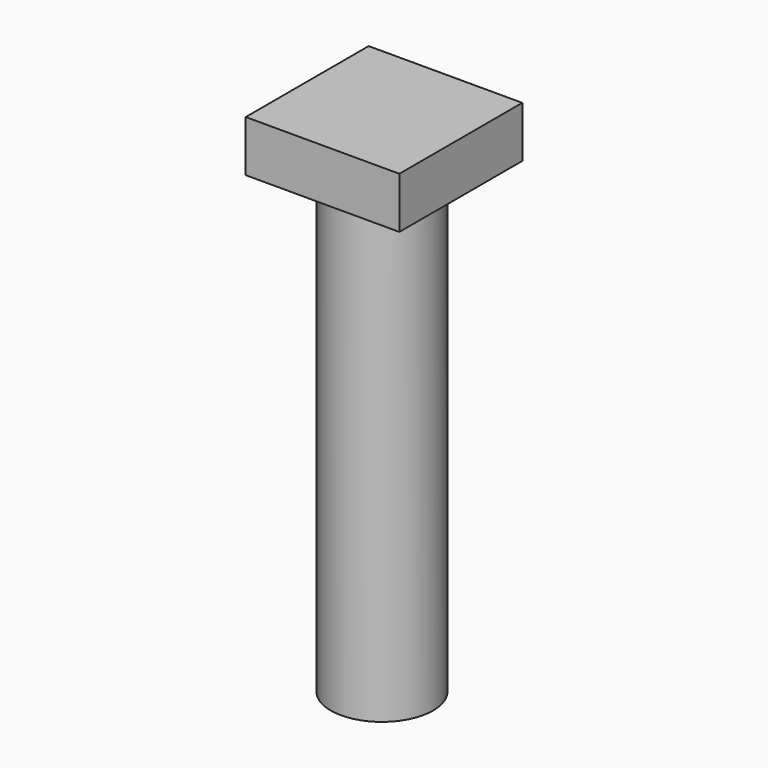
from build123d import *

# Parameters (mm, degrees)
F0_W     = 7.62
F0_H     = 7.62
F1_DEPTH = 2.54
F2_R     = 1.27
F3_DEPTH = 22.86
F4_R     = 0.254
F5_DEPTH = 2.54
F2_R_2   = 2.54
F6_DEPTH = 22.86


# Not quite as in the source:
# - a feature names something its author has since deleted; it is built from what else it names


with BuildPart() as f1:
    # F0 (on Top) → F1 (new body)
    with BuildSketch(Plane.XY):
        with Locations((-38.7955456972, -21.8359371471)):
            Rectangle(F0_W, F0_H)
    extrude(amount=F1_DEPTH)

    # F2 (on face) → F3 (join)
    with BuildSketch(Plane(origin=(0, 0, 0), x_dir=(1, 0, 0), z_dir=(0, 0, -1))):
        with Locations((-38.854431361, 21.8882076442)):
            Circle(F2_R)
    extrude(amount=F3_DEPTH)

    # F4 (on face) → F5 (cut)
    with BuildSketch(Plane(origin=(0, 0, -22.86), x_dir=(1, 0, 0), z_dir=(0, 0, -1))):
        with Locations((-38.854431361, 21.8882076442)):
            Circle(F4_R)
    extrude(amount=-F5_DEPTH, mode=Mode.SUBTRACT)

    # F2 (on face) → F6 (join)
    with BuildSketch(Plane(origin=(0, 0, 0), x_dir=(1, 0, 0), z_dir=(0, 0, -1))):
        with Locations((-38.854431361, 21.8882076442)):
            Circle(F2_R_2)
        with Locations((-38.854431361, 21.8882076442)):
            Circle(F2_R, mode=Mode.SUBTRACT)
    extrude(amount=F6_DEPTH)


solid = f1.part
